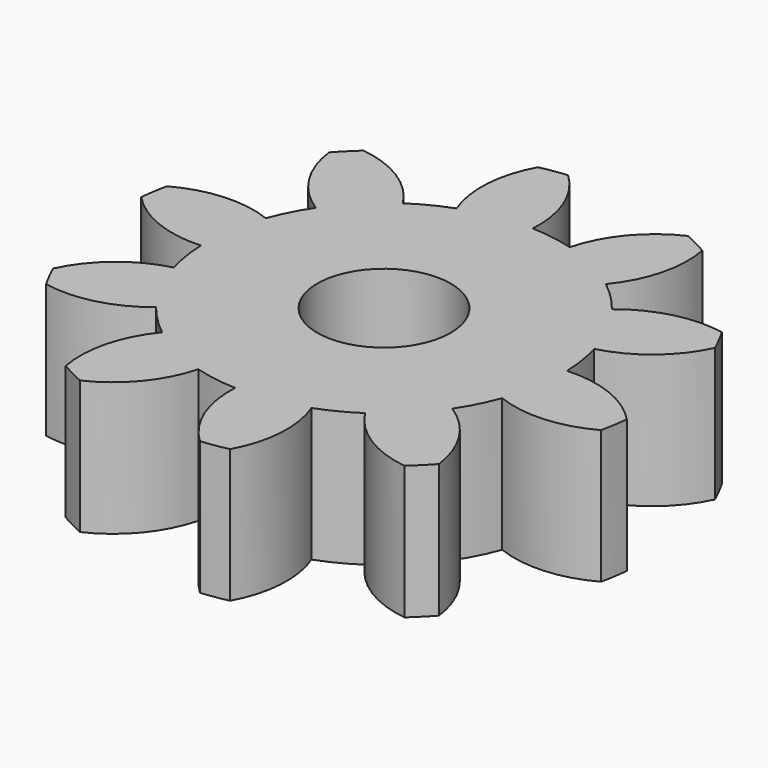
from build123d import *

# Parameters (mm, degrees)
F0_R            = 3.175
F1_DEPTH        = 6.35
F1_COPIES_COUNT = 10


# Not quite as in the source:
# - a feature of the source that left no trace in its solid (it failed there, or was rolled back) is left out
# - a pattern or mirror of a feature is missing from the dataset's text; its kind, count and spacing are read off the source's solid


with BuildPart() as f1:
    # F0 (on Top) → F1 (new body)
    with BuildSketch(Plane.XY):
        with BuildLine():
            ThreePointArc((-2.909315706, 7.9511210887), (-4.8503730853, -6.9396199736), (8.4666666667, 0))
            ThreePointArc((8.4666666667, 0), (6.0954162172, 5.8762526821), (0.3098921194, 8.4609935184))
            ThreePointArc((0.3098921194, 8.4609935184), (-1.3244784707, 8.3624279504), (-2.909315706, 7.9511210887))
        make_face()
        Circle(F0_R, mode=Mode.SUBTRACT)
        with BuildLine():
            ThreePointArc((-2.909315706, 7.9511210887), (-1.3244784707, 8.3624279504), (0.3098921194, 8.4609935184))
            ThreePointArc((0.3098921194, 8.4609935184), (-0.0554250299, 10.7289090003), (-1.3473672642, 12.6283253623))
            ThreePointArc((-1.3473672642, 12.6283253623), (-1.986717706, 12.5436419256), (-2.620944731, 12.426610508))
            ThreePointArc((-2.620944731, 12.426610508), (-3.2627028763, 10.2209260937), (-2.909315706, 7.9511210887))
        make_face()
    extrude(amount=F1_DEPTH)

    # F1_copies: F1 ×10 about axis
    f1_copies_axis = Axis((0, 0, 0), (0, 0, 1))


with BuildPart() as f1_1:
    add(f1.part)
    for i in range(1, F1_COPIES_COUNT):
        add(f1.part.rotate(f1_copies_axis, i * 360 / F1_COPIES_COUNT))


solid = f1_1.part
